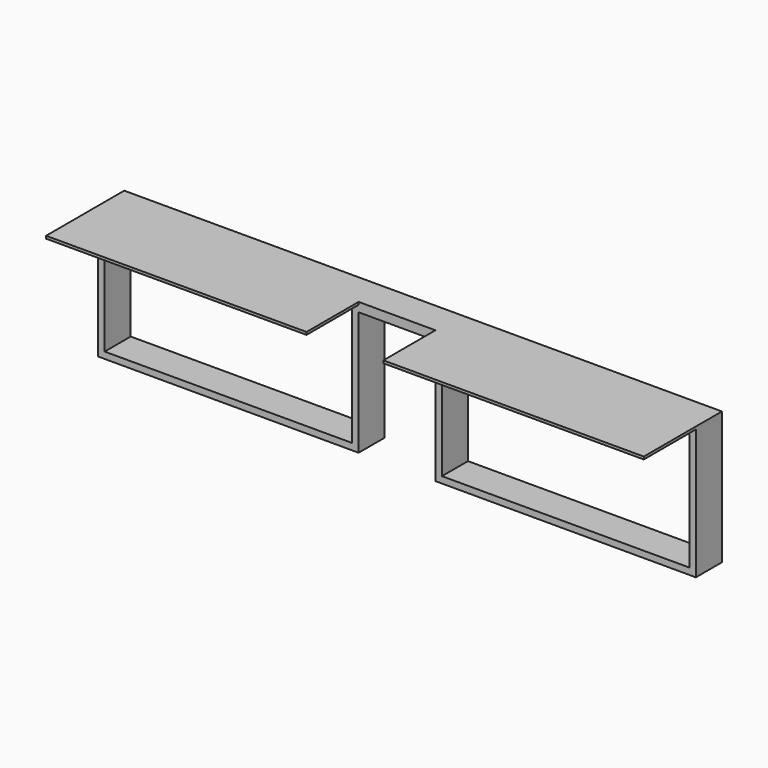
from build123d import *

# Parameters (mm, degrees)
F0_W     = 14.986
F0_H     = 1.27
F1_DEPTH = 1.27
F0_W_2   = 48.26
F0_H_2   = 22.86
F2_DEPTH = 6.35
F3_W     = 50.8
F3_H     = 12.7
F4_DEPTH = 0.508


# Not quite as in the source:
# - a feature names something its author has since deleted; it is built from what else it names


with BuildPart() as f1:
    # F0 (on Front) → F1 (new body)
    with BuildSketch(Plane.XZ):
        with Locations((-7.493, 49.4207651077)):
            Rectangle(F0_W, F0_H)
    extrude(amount=F1_DEPTH)

    # F0 (on Front) → F2 (join)
    with BuildSketch(Plane.XZ):
        Polygon((-14.986, 50.0557651077), (-65.786, 50.0557651077), (-65.786, 24.6557651077), (-14.986, 24.6557651077), (-14.986, 34.8157651077), (-14.986, 48.7857651077), align=None)
        with Locations((-40.386, 37.3557651077)):
            Rectangle(F0_W_2, F0_H_2, mode=Mode.SUBTRACT)
        with Locations((-7.493, 49.4207651077)):
            Rectangle(F0_W, F0_H)
        Polygon((50.8, 50.0557651077), (0, 50.0557651077), (0, 48.7857651077), (0, 34.8157651077), (0, 24.6557651077), (50.8, 24.6557651077), align=None)
        with Locations((25.4, 37.3557651077)):
            Rectangle(F0_W_2, F0_H_2, mode=Mode.SUBTRACT)
    extrude(amount=F2_DEPTH)

    # F3 (on face) → F4 (join)
    with BuildSketch(Plane.XY.offset(50.0557651077)):
        with Locations((-40.386, -12.7)):
            Rectangle(F3_W, F3_H)
        with Locations((25.4, -12.7)):
            Rectangle(F3_W, F3_H)
        Polygon((-65.786, 0), (-65.786, -6.35), (-14.986, -6.35), (0, -6.35), (50.8, -6.35), (50.8, 0), align=None)
    extrude(amount=F4_DEPTH)


solid = f1.part
